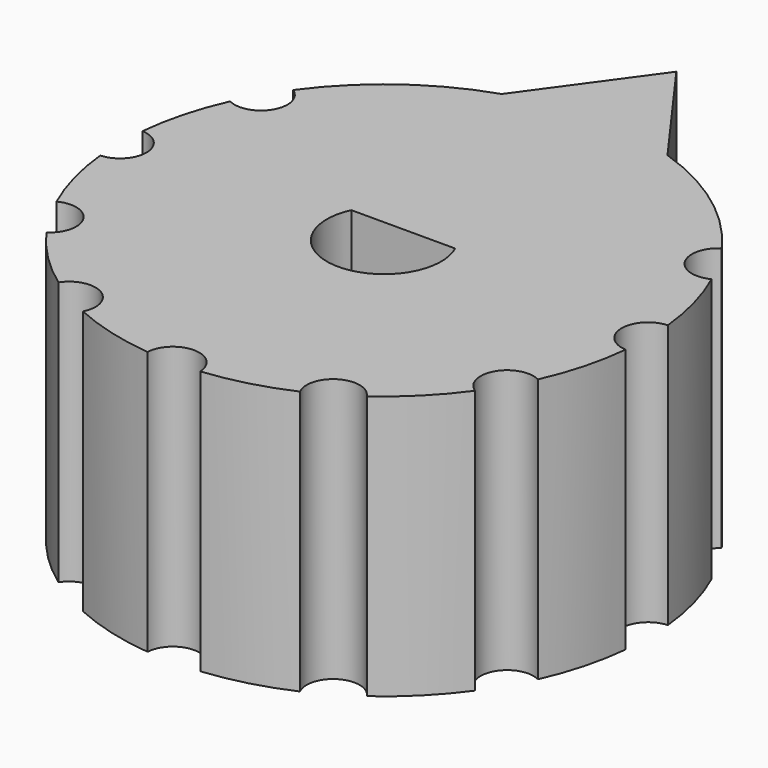
from build123d import *

# Parameters (mm, degrees)
F0_R     = 15
F1_DEPTH = 10
F2_R     = 15
F3_DEPTH = 5
F5_DEPTH = 15
F6_DEPTH = 15


# Not quite as in the source:
# - a feature names something its author has since deleted; it is built from what else it names


with BuildPart() as f1:
    # F0 (on Top) → F1 (new body)
    with BuildSketch(Plane.XY):
        Circle(F0_R)
        with BuildLine():
            ThreePointArc((2.9510768453, 1.3614864865), (0, -3.25), (-2.9510768453, 1.3614864865))
            Line((-2.9510768453, 1.3614864865), (2.9510768453, 1.3614864865))
        make_face(mode=Mode.SUBTRACT)
    extrude(amount=F1_DEPTH)

    # F2 (on face) → F3 (join)
    with BuildSketch(Plane(origin=(0, 0, 0), x_dir=(1, 0, 0), z_dir=(0, 0, -1))):
        Circle(F2_R)
        with BuildLine():
            ThreePointArc((-2.9510768453, -1.3614864865), (0, 3.25), (2.9510768453, -1.3614864865))
            Line((2.9510768453, -1.3614864865), (-2.9510768453, -1.3614864865))
        make_face(mode=Mode.SUBTRACT)
        with BuildLine():
            Line((-2.9510768453, -1.3614864865), (2.9510768453, -1.3614864865))
            ThreePointArc((2.9510768453, -1.3614864865), (0, 3.25), (-2.9510768453, -1.3614864865))
        make_face()
    extrude(amount=F3_DEPTH)

    # F4 (on face) → F5 (join)
    with BuildSketch(Plane.XY.offset(10)):
        with BuildLine():
            Line((4.707880128, 14.2420456642), (0, 20.7567233592))
            Line((0, 20.7567233592), (-4.707880128, 14.2420456642))
            ThreePointArc((-4.707880128, 14.2420456642), (0, 15), (4.707880128, 14.2420456642))
        make_face()
    extrude(amount=-F5_DEPTH)

    # F4 (on face) → F6 (cut, through all)
    with BuildSketch(Plane.XY.offset(10)):
        with BuildLine():
            ThreePointArc((13.6744910648, 6.1650867081), (12.9903810568, 7.5), (12.1763672382, 8.7599132919))
            ThreePointArc((12.1763672382, 8.7599132919), (11.6913429511, 6.75), (13.6744910648, 6.1650867081))
        make_face()
        with BuildLine():
            ThreePointArc((15, 0), (14.9812382666, 0.75), (14.925, 1.4981238267))
            ThreePointArc((14.925, 1.4981238267), (13.5, 0), (14.925, -1.4981238267))
            ThreePointArc((14.925, -1.4981238267), (14.9812382666, -0.75), (15, 0))
        make_face()
        with BuildLine():
            ThreePointArc((12.1763672382, -8.7599132919), (12.9903810568, -7.5), (13.6744910648, -6.1650867081))
            ThreePointArc((13.6744910648, -6.1650867081), (11.6913429511, -6.75), (12.1763672382, -8.7599132919))
        make_face()
        with BuildLine():
            ThreePointArc((6.1650867081, -13.6744910648), (7.5, -12.9903810568), (8.7599132919, -12.1763672382))
            ThreePointArc((8.7599132919, -12.1763672382), (6.75, -11.6913429511), (6.1650867081, -13.6744910648))
        make_face()
        with BuildLine():
            ThreePointArc((1.4981238267, -14.925), (0, -13.5), (-1.4981238267, -14.925))
            ThreePointArc((-1.4981238267, -14.925), (0, -15), (1.4981238267, -14.925))
        make_face()
        with BuildLine():
            ThreePointArc((-6.1650867081, -13.6744910648), (-6.75, -11.6913429511), (-8.7599132919, -12.1763672382))
            ThreePointArc((-8.7599132919, -12.1763672382), (-7.5, -12.9903810568), (-6.1650867081, -13.6744910648))
        make_face()
        with BuildLine():
            ThreePointArc((-12.1763672382, -8.7599132919), (-11.6913429511, -6.75), (-13.6744910648, -6.1650867081))
            ThreePointArc((-13.6744910648, -6.1650867081), (-12.9903810568, -7.5), (-12.1763672382, -8.7599132919))
        make_face()
        with BuildLine():
            ThreePointArc((-14.925, -1.4981238267), (-13.5, 0), (-14.925, 1.4981238267))
            ThreePointArc((-14.925, 1.4981238267), (-15, 0), (-14.925, -1.4981238267))
        make_face()
        with BuildLine():
            ThreePointArc((-13.6744910648, 6.1650867081), (-11.6913429511, 6.75), (-12.1763672382, 8.7599132919))
            ThreePointArc((-12.1763672382, 8.7599132919), (-12.9903810568, 7.5), (-13.6744910648, 6.1650867081))
        make_face()
    extrude(amount=-F6_DEPTH, mode=Mode.SUBTRACT)


solid = f1.part
